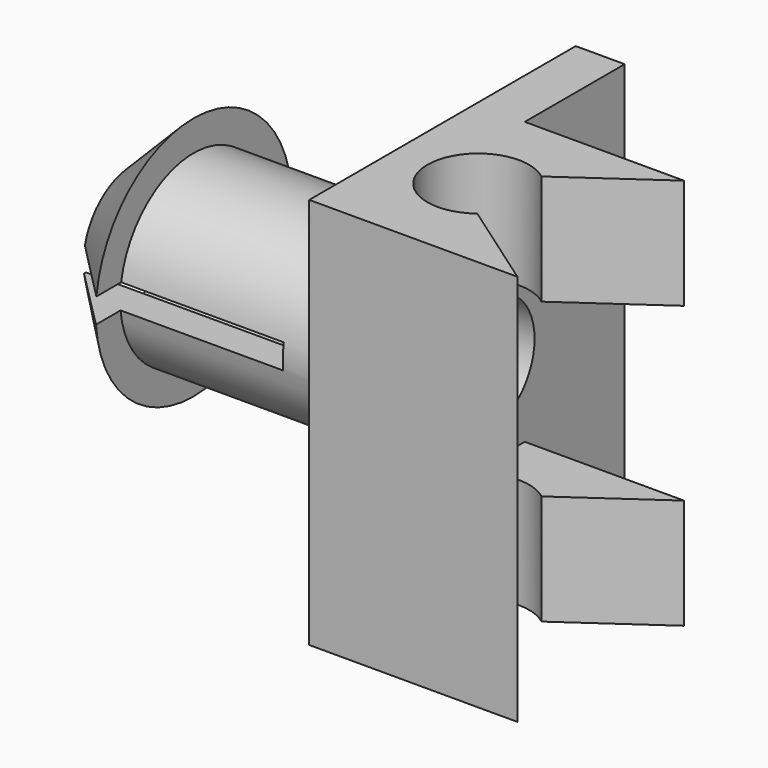
from build123d import *

# Parameters (mm, degrees)
F1_DEPTH  = 16
F2_W      = 6.5
F2_H      = 7
F3_DEPTH  = 6.5
F4_R      = 3.75
F4_R_2    = 2.4
F5_DEPTH  = 10
F6_DEPTH  = 8
F7_R      = 5
F8_DEPTH  = 2.5
F9_DEPTH  = 5
F10_SIZE2 = 2.49999
F10_SIZE  = 2.49999
F11_W     = 9.2321852261
F11_H     = 1
F12_DEPTH = 25


# Not quite as in the source:
# - a fillet or chamfer is up to 0.001 mm smaller than in the source, because OpenCascade refuses the exact size


with BuildPart() as f1:
    # F0 (on Top) → F1 (new body)
    with BuildSketch(Plane.XY):
        with BuildLine():
            Line((2, 13.6), (0, 13.6))
            Line((0, 13.6), (0, 0))
            Line((0, 0), (8.5, 0))
            Line((8.5, 0), (4.7718484698, 2.610479805))
            ThreePointArc((4.7718484698, 2.610479805), (1.425, 4.25), (4.7718484698, 5.889520195))
            Line((4.7718484698, 5.889520195), (8.5, 8.5))
            Line((8.5, 8.5), (2, 8.5))
            Line((2, 8.5), (2, 13.6))
        make_face()
    extrude(amount=F1_DEPTH)

    # F2 (on face) → F3 (cut)
    with BuildSketch(Plane(origin=(0, 8.5, 0), x_dir=(-1, 0, 0), z_dir=(0, 1, 0))):
        with Locations((-5.25, 8)):
            Rectangle(F2_W, F2_H)
    extrude(amount=-F3_DEPTH, mode=Mode.SUBTRACT)

    # F4 (on face) → F5 (join)
    with BuildSketch(Plane(origin=(0, 0, 0), x_dir=(0, -1, 0), z_dir=(-1, 0, 0))):
        with Locations((-6.6, 8)):
            Circle(F4_R)
        with Locations((-6.6, 8)):
            Circle(F4_R_2, mode=Mode.SUBTRACT)
    extrude(amount=F5_DEPTH)

    # F6 (cut): a face of the model
    f6_faces = [f1.faces().sort_by_distance(p)[0] for p in [
        (0, 6.6, 8),
    ]]
    extrude(f6_faces, amount=-F6_DEPTH, mode=Mode.SUBTRACT)

    # F7 (on face) → F8 (join)
    with BuildSketch(Plane(origin=(-10, 0, 0), x_dir=(0, -1, 0), z_dir=(-1, 0, 0))):
        with Locations((-6.6, 8)):
            Circle(F7_R)
    extrude(amount=F8_DEPTH)

    # F9 (cut): a face of the model
    f9_faces = [f1.faces().sort_by_distance(p)[0] for p in [
        (-10, 6.6, 8),
    ]]
    extrude(f9_faces, amount=-F9_DEPTH, mode=Mode.SUBTRACT)

    # F10 (size 2.5 and 2.5 in the source; OpenCascade refuses exactly that, so slightly less here)
    f10_edges = [f1.edges().sort_by_distance(p)[0] for p in [
        (-12.5, 11.6, 8),
    ]]
    chamfer(f10_edges, length=F10_SIZE, length2=F10_SIZE2)

    # F11 (on face) → F12 (cut)
    with BuildSketch(Plane(origin=(0, 13.6, 0), x_dir=(-1, 0, 0), z_dir=(0, 1, 0))):
        with Locations((7.9738140339, 8.1086927094)):
            Rectangle(F11_W, F11_H)
    extrude(amount=-F12_DEPTH, mode=Mode.SUBTRACT)


solid = f1.part
